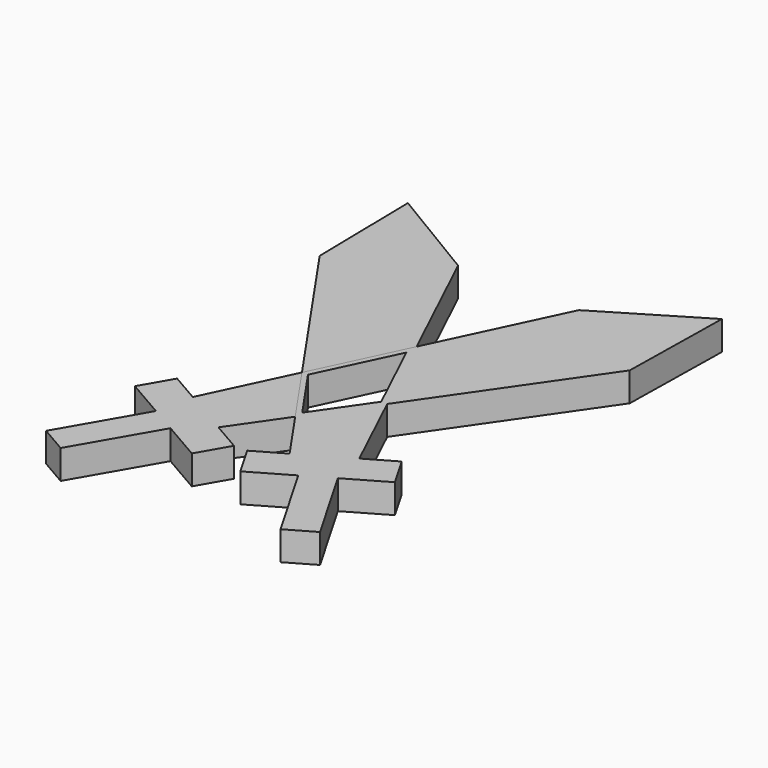
from build123d import *

# Parameters (mm, degrees)
F1_DEPTH = 5.08
F2_DEPTH = 5.08
F3_DEPTH = 5.08
F4_DEPTH = 5.08
F5_DEPTH = 5.08
F6_DEPTH = 5.08
F7_DEPTH = 5.08
F8_DEPTH = 5.08
F9_DEPTH = 5.08


with BuildPart() as f1:
    # F0 (on Top) → F1 (new body)
    with BuildSketch(Plane.XY):
        Polygon((-27.1429486431, 27.5143728866), (-7.4663818198, -0.961395638), (0, 14.7941357478), (-10.5639939546, 37.0862368388), (-27.4876418162, 47.2551268799), align=None)
    extrude(amount=F1_DEPTH)


with BuildPart() as f2:
    # F0 (on Top) → F2 (new body)
    with BuildSketch(Plane.XY):
        Polygon((-7.4663818198, -0.961395638), (-14.5768045919, -15.965783554), (-6.231049466, -20.7842075226), (0, -11.7666830809), align=None)
    extrude(amount=F2_DEPTH)

    # F0 (on Top) → F7 (join)
    with BuildSketch(Plane.XY):
        Polygon((-19.660384601, -13.0307772673), (-22.7609974951, -18.4011963345), (-15.9242138402, -22.348415218), (-11.1885193949, -25.0825696808), (-4.248082351, -29.0896328764), (-1.1474694569, -23.7192138093), (-6.231049466, -20.7842075226), (-14.5768045919, -15.965783554), align=None)
    extrude(amount=F7_DEPTH)

    # F0 (on Top) → F8 (join)
    with BuildSketch(Plane.XY):
        Polygon((-11.1885193949, -25.0825696808), (-15.9242138402, -22.348415218), (-23.9827748524, -36.3062523269), (-19.2470804071, -39.0404067898), align=None)
    extrude(amount=F8_DEPTH)


with BuildPart() as f3:
    # F0 (on Top) → F3 (new body)
    with BuildSketch(Plane.XY):
        Polygon((0, 14.7941357478), (-7.4663818198, -0.961395638), (0, -11.7666830809), (7.4663818198, -0.961395638), align=None)
        Polygon((-6.4083149498, -0.961395638), (0, 12.5614069402), (6.4083149498, -0.961395638), (0, -10.2354572557), align=None, mode=Mode.SUBTRACT)
    extrude(amount=F3_DEPTH)

    # F0 (on Top) → F4 (join)
    with BuildSketch(Plane.XY):
        Polygon((10.5639939546, 37.0862368388), (0, 14.7941357478), (7.4663818198, -0.961395638), (27.1429486431, 27.5143728866), (27.4876418162, 47.2551268799), align=None)
    extrude(amount=F4_DEPTH)

    # F0 (on Top) → F5 (join)
    with BuildSketch(Plane.XY):
        Polygon((7.4663818198, -0.961395638), (0, -11.7666830809), (6.231049466, -20.7842075226), (14.5768045919, -15.965783554), align=None)
    extrude(amount=F5_DEPTH)

    # F0 (on Top) → F6 (join)
    with BuildSketch(Plane.XY):
        Polygon((14.5768045919, -15.965783554), (6.231049466, -20.7842075226), (1.1474694569, -23.7192138093), (4.248082351, -29.0896328764), (11.1885193949, -25.0825696808), (15.9242138402, -22.348415218), (22.7609974951, -18.4011963345), (19.660384601, -13.0307772673), align=None)
    extrude(amount=F6_DEPTH)

    # F0 (on Top) → F9 (join)
    with BuildSketch(Plane.XY):
        Polygon((15.9242138402, -22.348415218), (11.1885193949, -25.0825696808), (19.2470804071, -39.0404067898), (23.9827748524, -36.3062523269), align=None)
    extrude(amount=F9_DEPTH)


solid = Compound([f1.part, f2.part, f3.part])
